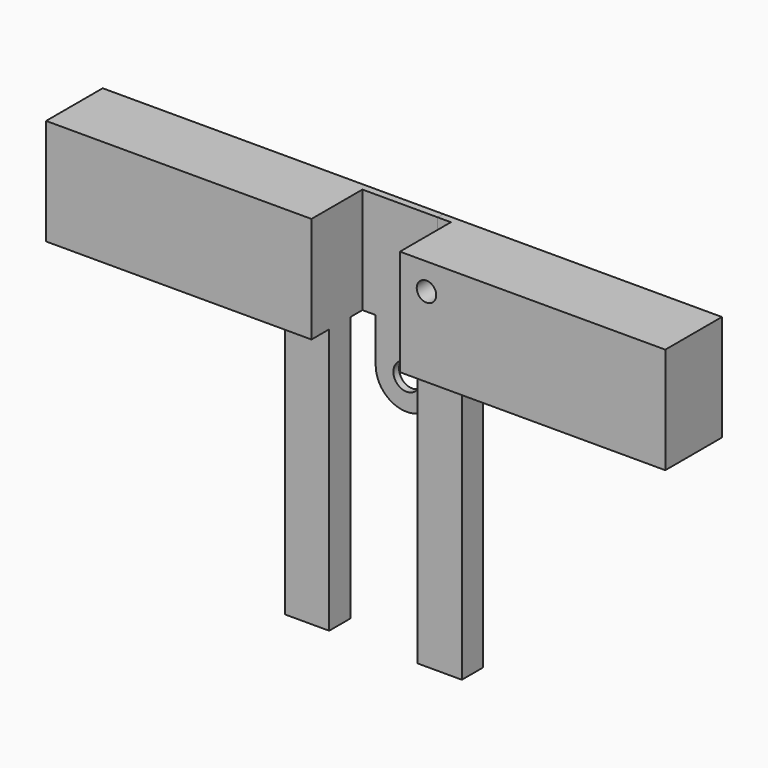
from build123d import *

# Parameters (mm, degrees)
F0_W     = 150
F0_H     = 60
F1_DEPTH = 20
F2_W     = 25
F2_H     = 150
F3_DEPTH = 7.5
F4_R     = 7.5
F5_DEPTH = 4
F6_R     = 5.5
F7_DEPTH = 40.001
F8_R     = 7.5
F9_DEPTH = 4


with BuildPart() as f1:
    # F0 (on Front) → F1 (new body, symmetric)
    with BuildSketch(Plane.XZ):
        with Locations((100, 0)):
            Rectangle(F0_W, F0_H)
    extrude(amount=F1_DEPTH, both=True)

    # F2 (on Front) → F3, piece 2 (join, symmetric)
    with BuildSketch(Plane.XZ):
        with Locations((37.5, -105)):
            Rectangle(F2_W, F2_H)
    extrude(amount=F3_DEPTH, both=True)

    # F6 (on face) → F7 (cut, through all)
    with BuildSketch(Plane(origin=(0, 20, 0), x_dir=(-1, 0, 0), z_dir=(0, 1, 0))):
        with Locations((-40, 15)):
            Circle(F6_R)
    extrude(amount=-F7_DEPTH, mode=Mode.SUBTRACT)

    # F8 (on face) → F9 (join)
    with BuildSketch(Plane(origin=(0, 20, 0), x_dir=(-1, 0, 0), z_dir=(0, 1, 0))):
        with BuildLine():
            Line((-17.5, 30), (-25, 30))
            Line((-25, 30), (-25, -30))
            Line((-25, -30), (-17.5, -30))
            Line((-17.5, -30), (-17.5, -55))
            ThreePointArc((-17.5, -55), (0, -37.5), (17.5, -55))
            Line((17.5, -55), (17.5, 30))
            Line((17.5, 30), (-17.5, 30))
        make_face()
        with BuildLine():
            ThreePointArc((-17.5, -55), (0, -72.5), (17.5, -55))
            ThreePointArc((17.5, -55), (0, -37.5), (-17.5, -55))
        make_face()
        with Locations((0, -55)):
            Circle(F8_R, mode=Mode.SUBTRACT)
    extrude(amount=-F9_DEPTH)


with BuildPart() as f1b:
    # F0 (on Front) → F1, piece 2 (new body, symmetric)
    with BuildSketch(Plane.XZ):
        with Locations((-100, 0)):
            Rectangle(F0_W, F0_H)
    extrude(amount=F1_DEPTH, both=True)

    # F2 (on Front) → F3 (join, symmetric)
    with BuildSketch(Plane.XZ):
        with Locations((-37.5, -105)):
            Rectangle(F2_W, F2_H)
    extrude(amount=F3_DEPTH, both=True)

    # F4 (on face) → F5 (join)
    with BuildSketch(Plane(origin=(0, 20, 0), x_dir=(-1, 0, 0), z_dir=(0, 1, 0))):
        with BuildLine():
            Line((25, 30), (17.5, 30))
            Line((17.5, 30), (-17.5, 30))
            Line((-17.5, 30), (-17.5, -55))
            ThreePointArc((-17.5, -55), (0, -37.5), (17.5, -55))
            Line((17.5, -55), (17.5, -30))
            Line((17.5, -30), (25, -30))
            Line((25, -30), (25, 30))
        make_face()
        with BuildLine():
            ThreePointArc((17.5, -55), (0, -37.5), (-17.5, -55))
            ThreePointArc((-17.5, -55), (0, -72.5), (17.5, -55))
        make_face()
        with Locations((0, -55)):
            Circle(F4_R, mode=Mode.SUBTRACT)
    extrude(amount=-F5_DEPTH)


solid = Compound([f1.part, f1b.part])
